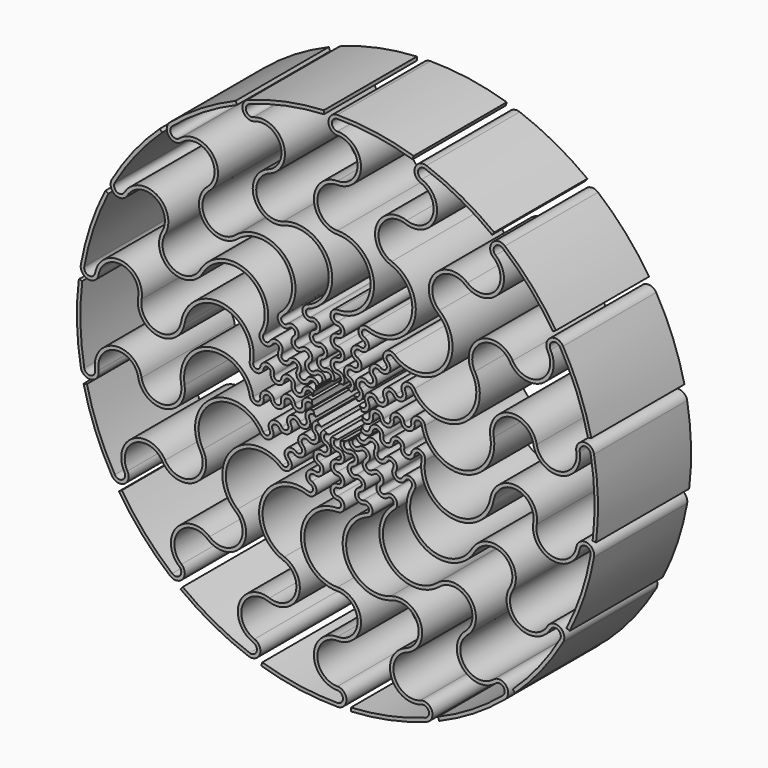
from build123d import *

# Parameters (mm, degrees)
F1_DEPTH        = 50.8
F1_COPIES_COUNT = 18


# Not quite as in the source:
# - ends of sketch curves that miss each other by under 0.0002 mm in the source are joined
# - a pattern or mirror of a feature is missing from the dataset's text; its kind, count and spacing are read off the source's solid


with BuildPart() as f1:
    # F0 (on Front) → F1 (new body)
    with BuildSketch(Plane.XZ):
        with BuildLine():
            ThreePointArc((0, 20.32), (-3.07975, 17.24025), (0, 14.1605))
            ThreePointArc((0, 14.1605), (1.55575, 12.60475), (0, 11.049))
            ThreePointArc((0, 11.049), (1.2442428961, 10.9787185325), (2.4726568092, 10.7687682352))
            ThreePointArc((2.4726568092, 10.7687682352), (2.7512929486, 13.9886747985), (0, 15.6845001095))
            ThreePointArc((0, 15.6845001095), (-1.5557498905, 17.24025), (0, 18.7959998905))
            ThreePointArc((0, 18.7959998905), (3.0797501095, 21.87575), (0, 24.9555001095))
            ThreePointArc((0, 24.9555001095), (-1.5557498905, 26.51125), (0, 28.0669998905))
            ThreePointArc((0, 28.0669998905), (3.0797501095, 31.14675), (0, 34.2265001095))
            ThreePointArc((0, 34.2265001095), (-1.5557498905, 35.78225), (0, 37.3379998905))
            ThreePointArc((0, 37.3379998905), (15.9721396226, 53.3101395131), (0, 69.2822791357))
            ThreePointArc((0, 69.2822791357), (-8.7629998905, 78.0452790263), (0, 86.8082789168))
            ThreePointArc((0, 86.8082789168), (10.2870001095, 97.0952790263), (0, 107.3822791357))
            ThreePointArc((0, 107.3822791357), (-2.4129998905, 109.7952790263), (0, 112.2082789168))
            ThreePointArc((0, 112.2082789168), (16.5854394216, 110.9757664511), (32.8065253776, 107.3053094346))
            Line((32.8065253776, 107.3053094346), (33.2521003009, 108.7627193393))
            ThreePointArc((33.2521003009, 108.7627193393), (16.8107011893, 112.4830281333), (0, 113.7322790263))
            ThreePointArc((0, 113.7322790263), (-3.937, 109.7952790263), (0, 105.8582790263))
            ThreePointArc((0, 105.8582790263), (8.763, 97.0952790263), (0, 88.3322790263))
            ThreePointArc((0, 88.3322790263), (-10.287, 78.0452790263), (0, 67.7582790263))
            ThreePointArc((0, 67.7582790263), (14.4481395131, 53.3101395131), (0, 38.862))
            ThreePointArc((0, 38.862), (-3.07975, 35.78225), (0, 32.7025))
            ThreePointArc((0, 32.7025), (1.55575, 31.14675), (0, 29.591))
            ThreePointArc((0, 29.591), (-3.07975, 26.51125), (0, 23.4315))
            ThreePointArc((0, 23.4315), (1.55575, 21.87575), (0, 20.32))
        make_face()
    extrude(amount=F1_DEPTH)


with BuildPart() as f1_copies_1:
    # F1_copies: instance of F1
    add(f1.part.rotate(Axis((0, 0, 0), (0, 1, 0)), 1 * 360 / F1_COPIES_COUNT))


with BuildPart() as f1_copies_2:
    # F1_copies: instance of F1
    add(f1.part.rotate(Axis((0, 0, 0), (0, 1, 0)), 2 * 360 / F1_COPIES_COUNT))


with BuildPart() as f1_copies_3:
    # F1_copies: instance of F1
    add(f1.part.rotate(Axis((0, 0, 0), (0, 1, 0)), 3 * 360 / F1_COPIES_COUNT))


with BuildPart() as f1_copies_4:
    # F1_copies: instance of F1
    add(f1.part.rotate(Axis((0, 0, 0), (0, 1, 0)), 4 * 360 / F1_COPIES_COUNT))


with BuildPart() as f1_copies_5:
    # F1_copies: instance of F1
    add(f1.part.rotate(Axis((0, 0, 0), (0, 1, 0)), 5 * 360 / F1_COPIES_COUNT))


with BuildPart() as f1_copies_6:
    # F1_copies: instance of F1
    add(f1.part.rotate(Axis((0, 0, 0), (0, 1, 0)), 6 * 360 / F1_COPIES_COUNT))


with BuildPart() as f1_copies_7:
    # F1_copies: instance of F1
    add(f1.part.rotate(Axis((0, 0, 0), (0, 1, 0)), 7 * 360 / F1_COPIES_COUNT))


with BuildPart() as f1_copies_8:
    # F1_copies: instance of F1
    add(f1.part.rotate(Axis((0, 0, 0), (0, 1, 0)), 8 * 360 / F1_COPIES_COUNT))


with BuildPart() as f1_copies_9:
    # F1_copies: instance of F1
    add(f1.part.rotate(Axis((0, 0, 0), (0, 1, 0)), 9 * 360 / F1_COPIES_COUNT))


with BuildPart() as f1_copies_10:
    # F1_copies: instance of F1
    add(f1.part.rotate(Axis((0, 0, 0), (0, 1, 0)), 10 * 360 / F1_COPIES_COUNT))


with BuildPart() as f1_copies_11:
    # F1_copies: instance of F1
    add(f1.part.rotate(Axis((0, 0, 0), (0, 1, 0)), 11 * 360 / F1_COPIES_COUNT))


with BuildPart() as f1_copies_12:
    # F1_copies: instance of F1
    add(f1.part.rotate(Axis((0, 0, 0), (0, 1, 0)), 12 * 360 / F1_COPIES_COUNT))


with BuildPart() as f1_copies_13:
    # F1_copies: instance of F1
    add(f1.part.rotate(Axis((0, 0, 0), (0, 1, 0)), 13 * 360 / F1_COPIES_COUNT))


with BuildPart() as f1_copies_14:
    # F1_copies: instance of F1
    add(f1.part.rotate(Axis((0, 0, 0), (0, 1, 0)), 14 * 360 / F1_COPIES_COUNT))


with BuildPart() as f1_copies_15:
    # F1_copies: instance of F1
    add(f1.part.rotate(Axis((0, 0, 0), (0, 1, 0)), 15 * 360 / F1_COPIES_COUNT))


with BuildPart() as f1_copies_16:
    # F1_copies: instance of F1
    add(f1.part.rotate(Axis((0, 0, 0), (0, 1, 0)), 16 * 360 / F1_COPIES_COUNT))


with BuildPart() as f1_copies_17:
    # F1_copies: instance of F1
    add(f1.part.rotate(Axis((0, 0, 0), (0, 1, 0)), 17 * 360 / F1_COPIES_COUNT))


solid = Compound([f1.part, f1_copies_1.part, f1_copies_2.part, f1_copies_3.part, f1_copies_4.part, f1_copies_5.part, f1_copies_6.part, f1_copies_7.part, f1_copies_8.part, f1_copies_9.part, f1_copies_10.part, f1_copies_11.part, f1_copies_12.part, f1_copies_13.part, f1_copies_14.part, f1_copies_15.part, f1_copies_16.part, f1_copies_17.part])
